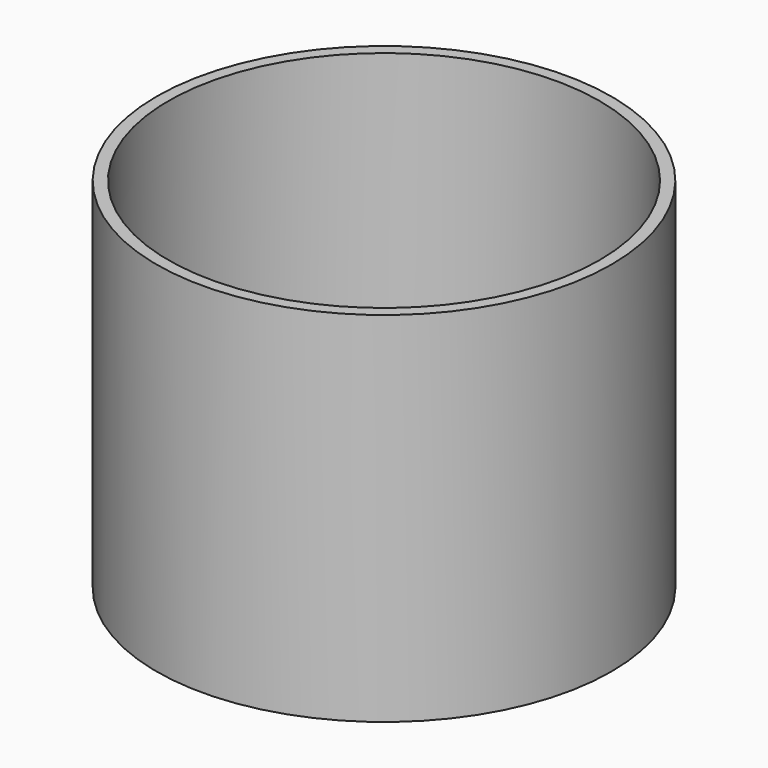
from build123d import *

# Parameters (mm, degrees)
F0_R     = 38.1
F0_R_2   = 36.1
F1_DEPTH = 60


# Not quite as in the source:
# - the program builds the solid bodies; features that only make, move or delete a surface that nothing else refers to are left out


with BuildPart() as f1:
    # F0 (on Top) → F1 (new body)
    with BuildSketch(Plane.XY):
        Circle(F0_R)
        Circle(F0_R_2, mode=Mode.SUBTRACT)
    extrude(amount=F1_DEPTH)


solid = f1.part
